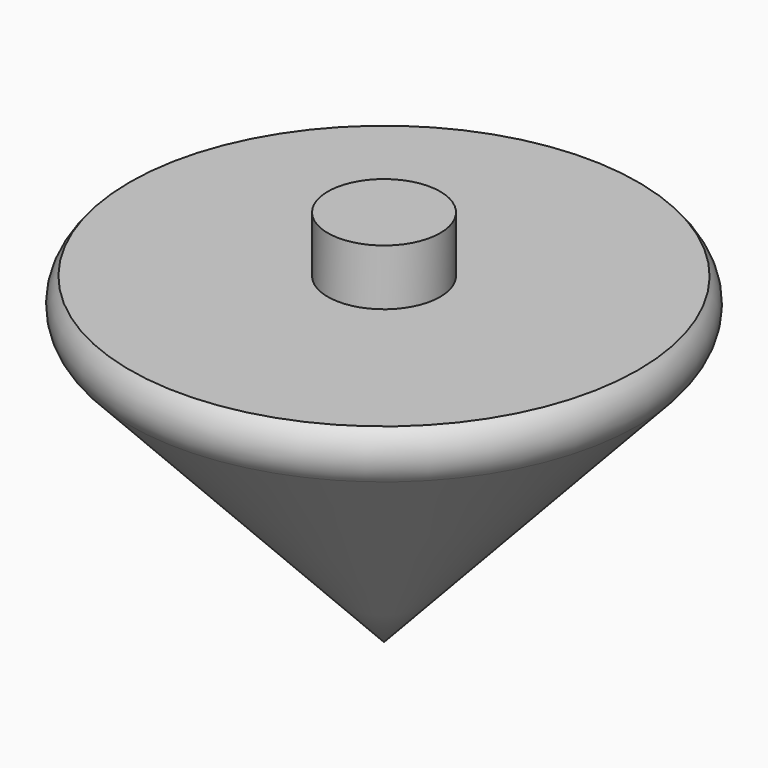
from build123d import *


# Not quite as in the source:
# - a feature names something its author has since deleted; it is built from what else it names


with BuildPart() as f1:
    # F0 (on Front) → F1 (revolve)
    with BuildSketch(Plane.XZ):
        with BuildLine():
            Line((0, 63.0670562387), (0, 0))
            Line((0, 0), (42.3725694418, 45.5658696592))
            ThreePointArc((42.3725694418, 45.5658696592), (43.9736000442, 49.6386233717), (42.3725694418, 53.7113770843))
            Line((42.3725694418, 53.7113770843), (9.3707125634, 53.7113770843))
            Line((9.3707125634, 53.7113770843), (9.3707125634, 63.0670562387))
            Line((9.3707125634, 63.0670562387), (0, 63.0670562387))
        make_face()
    revolve(axis=Axis((0, 0, 31.5335281193), (0, 0, 1)))


solid = f1.part
